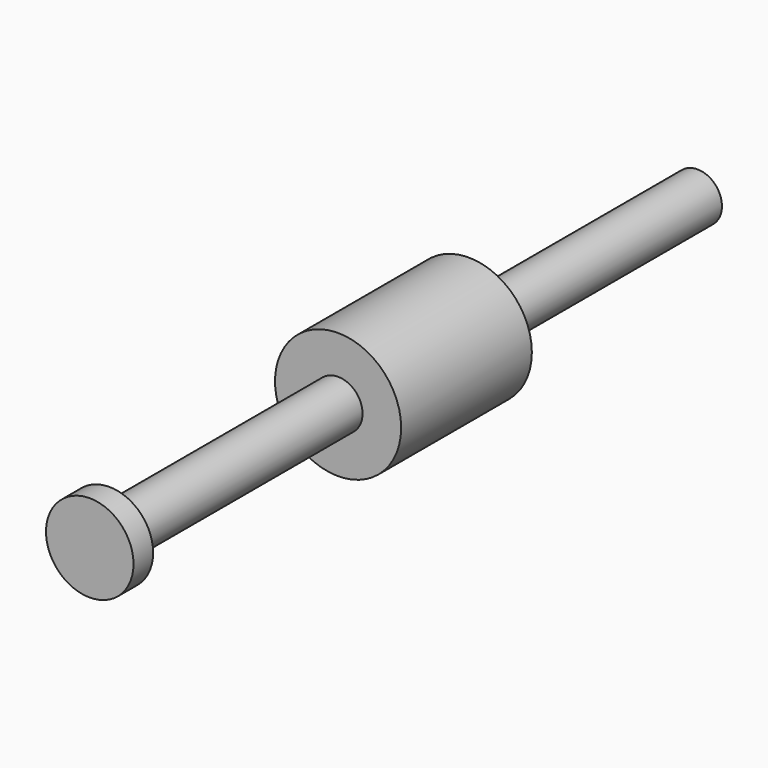
from build123d import *

# Parameters (mm, degrees)
F0_R     = 9.8054228033
F1_DEPTH = 25.4
F3_R     = 3.8049000848
F4_DEPTH = 44.45
F2_R     = 3.804929308
F5_DEPTH = 44.45
F6_R     = 6.8035972376
F7_DEPTH = 3.81


# Not quite as in the source:
# - a feature names something its author has since deleted; it is built from what else it names


with BuildPart() as f1:
    # F0 (on Front) → F1 (new body)
    with BuildSketch(Plane.XZ):
        Circle(F0_R)
    extrude(amount=F1_DEPTH)

    # F3 (on face) → F4 (join)
    with BuildSketch(Plane(origin=(0, 0, 0), x_dir=(-1, 0, 0), z_dir=(0, 1, 0))):
        Circle(F3_R)
    extrude(amount=F4_DEPTH)

    # F2 (on face) → F5 (join)
    with BuildSketch(Plane.XZ.offset(25.4)):
        Circle(F2_R)
    extrude(amount=F5_DEPTH)

    # F6 (on face) → F7 (join)
    with BuildSketch(Plane.XZ.offset(69.85)):
        Circle(F6_R)
    extrude(amount=F7_DEPTH)


solid = f1.part
